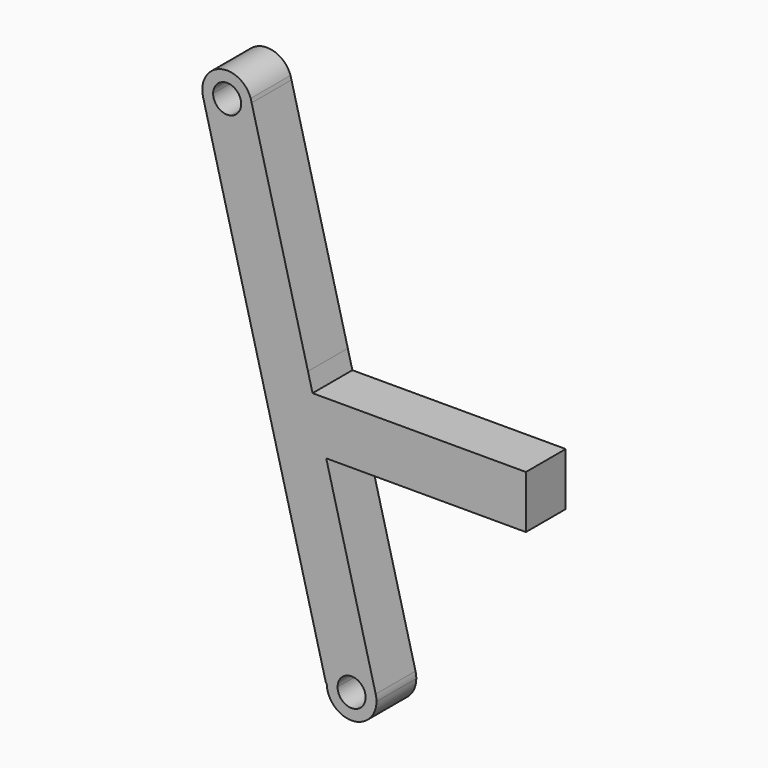
from build123d import *

# Parameters (mm, degrees)
F1_DEPTH = 25.4


# Not quite as in the source:
# - a feature names something its author has since deleted; it is built from what else it names


with BuildPart() as f1:
    # F0 (on Front) → F1 (new body)
    with BuildSketch(Plane.XZ):
        with BuildLine():
            ThreePointArc((-38.9001, 29.1195621888), (-31.75, 36.2696621888), (-24.5999, 29.1195621888))
            ThreePointArc((-24.5999, 29.1195621888), (-26.0973866941, 24.7409901814), (-29.9625922208, 22.1964773676))
            Line((-29.9625922208, 22.1964773676), (-28.5752082075, 16.8227863075))
            ThreePointArc((-28.5752082075, 16.8227863075), (-21.7098342702, 21.3423472555), (-19.05, 29.1195621888))
            ThreePointArc((-19.05, 29.1195621888), (-19.0991685805, 30.2360138876), (-19.2462936057, 31.3438208077))
            Line((-19.2462936057, 31.3438208077), (-19.7336528982, 33.2302071905))
            ThreePointArc((-19.7336528982, 33.2302071905), (-33.8335536719, 41.6474831694), (-44.45, 29.1195621888))
            Line((-44.45, 29.1195621888), (-38.9001, 29.1195621888))
        make_face()
        with BuildLine():
            ThreePointArc((-29.9625922208, 22.1964773676), (-36.1285720074, 23.4669488829), (-38.9001, 29.1195621888))
            Line((-38.9001, 29.1195621888), (-44.45, 29.1195621888))
            ThreePointArc((-44.45, 29.1195621888), (-44.3685455909, 27.683488663), (-44.1252272171, 26.2658363215))
            Line((-44.1252272171, 26.2658363215), (-43.9599962271, 25.6258546831))
            ThreePointArc((-43.9599962271, 25.6258546831), (-38.0573158317, 18.0965060336), (-28.5752082075, 16.8227863075))
            Line((-28.5752082075, 16.8227863075), (-29.9625922208, 22.1964773676))
        make_face()
        with BuildLine():
            Line((28.5710442304, -204.5191802253), (-28.5752082075, 16.8227863075))
            ThreePointArc((-28.5752082075, 16.8227863075), (-38.0573158317, 18.0965060336), (-43.9599962271, 25.6258546831))
            Line((-43.9599962271, 25.6258546831), (18.6335537415, -216.8148802954))
            Line((18.6335537415, -216.8148802954), (19.05, -216.8148802954))
            ThreePointArc((19.05, -216.8148802954), (21.7085175827, -209.039365466), (28.5710442304, -204.5191802253))
        make_face()
        with BuildLine():
            ThreePointArc((-19.05, 29.1195621888), (-21.7098342702, 21.3423472555), (-28.5752082075, 16.8227863075))
            Line((-28.5752082075, 16.8227863075), (28.5710442304, -204.5191802253))
            ThreePointArc((28.5710442304, -204.5191802253), (38.1974658289, -205.8732083763), (44.0462542776, -213.6380688845))
            Line((44.0462542776, -213.6380688845), (18.8073706418, -115.9477465067))
            Line((18.8073706418, -115.9477465067), (11.8328057084, -88.9518022083))
            Line((11.8328057084, -88.9518022083), (9.4897628664, -79.8827556578))
            Line((9.4897628664, -79.8827556578), (-19.2462936057, 31.3438208077))
            ThreePointArc((-19.2462936057, 31.3438208077), (-19.0991685805, 30.2360138876), (-19.05, 29.1195621888))
        make_face()
        with BuildLine():
            Line((29.958428385, -209.8928718327), (28.5710442304, -204.5191802253))
            ThreePointArc((28.5710442304, -204.5191802253), (21.7085175827, -209.039365466), (19.05, -216.8148802954))
            Line((19.05, -216.8148802954), (24.5999, -216.8148802954))
            ThreePointArc((24.5999, -216.8148802954), (26.0960701183, -212.4380084784), (29.958428385, -209.8928718327))
        make_face()
        with BuildLine():
            ThreePointArc((44.0462542776, -213.6380688845), (38.1974658289, -205.8732083763), (28.5710442304, -204.5191802253))
            Line((28.5710442304, -204.5191802253), (29.958428385, -209.8928718327))
            ThreePointArc((29.958428385, -209.8928718327), (36.126871817, -211.1609504137), (38.9001, -216.8148802954))
            ThreePointArc((38.9001, -216.8148802954), (37.4012962188, -221.1951520972), (33.5332432967, -223.7390389703))
            Line((33.5332432967, -223.7390389703), (34.9206274513, -229.1127305777))
            ThreePointArc((34.9206274513, -229.1127305777), (41.7888487545, -224.5937951095), (44.45, -216.8148802954))
            ThreePointArc((44.45, -216.8148802954), (44.3486592407, -215.2136978145), (44.0462542776, -213.6380688845))
        make_face()
        with BuildLine():
            Line((24.5999, -216.8148802954), (19.05, -216.8148802954))
            ThreePointArc((19.05, -216.8148802954), (19.1512093102, -218.4150281492), (19.4532241187, -219.9896720879))
            ThreePointArc((19.4532241187, -219.9896720879), (25.2979309254, -227.7538384111), (34.9206274513, -229.1127305777))
            Line((34.9206274513, -229.1127305777), (33.5332432967, -223.7390389703))
            ThreePointArc((33.5332432967, -223.7390389703), (27.3697281982, -222.4661765142), (24.5999, -216.8148802954))
        make_face()
        Polygon((11.8328057084, -88.9518022083), (18.8073706418, -115.9477465067), (120.7016461253, -115.9477465067), (120.7016461253, -88.9518022083), align=None)
    extrude(amount=F1_DEPTH)


solid = f1.part
